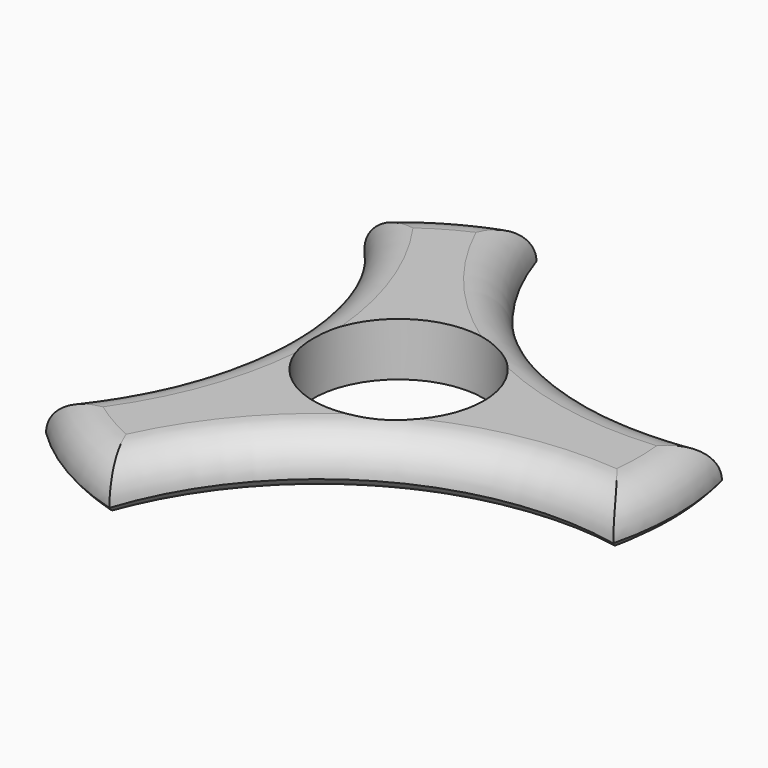
from build123d import *

# Parameters (mm, degrees)
F0_R         = 11.2
F1_DEPTH     = 7
F2_T2_ANGLE  = 120.2325245339
F2_T4_ANGLE  = 67.6545772904
F2_T6_ANGLE  = 120.2325245339
F2_T8_ANGLE  = 67.6545772904
F2_T10_ANGLE = 120.2325245339
F2_T12_ANGLE = 67.6545772904
F3_T2_ANGLE  = 112.9190333921
F3_T4_ANGLE  = 59.7918695457
F3_T6_ANGLE  = 112.9190333921
F3_T8_ANGLE  = 112.9190333921
F3_T10_ANGLE = 59.7918695457
F3_T12_ANGLE = 59.7918694889


# Not quite as in the source:
# - a fillet or chamfer that OpenCascade refuses, or shapes differently, is made with other operations: its cross-section is extruded or revolved along the edge and cut away or added


with BuildPart() as f1:
    # F0 (on Top) → F1 (new body)
    with BuildSketch(Plane.XY):
        with BuildLine():
            ThreePointArc((35.3273925443, 8.9196701012), (7.7000134584, 13.3368145289), (-9.9390353711, 35.0542544434))
            ThreePointArc((-9.9390353711, 35.0542544434), (-18.2180211514, 31.5545382476), (-25.3883571732, 26.1345843422))
            ThreePointArc((-25.3883571732, 26.1345843422), (-15.4000269168, 0), (-25.3883571732, -26.1345843422))
            ThreePointArc((-25.3883571732, -26.1345843422), (-18.2180211514, -31.5545382476), (-9.9390353711, -35.0542544434))
            ThreePointArc((-9.9390353711, -35.0542544434), (7.7000134584, -13.3368145289), (35.3273925443, -8.9196701012))
            ThreePointArc((35.3273925443, -8.9196701012), (36.4360423028, 0), (35.3273925443, 8.9196701012))
        make_face()
        Circle(F0_R, mode=Mode.SUBTRACT)
    extrude(amount=F1_DEPTH)

    # F2: fillet of radius 5 on 6 edges, made by hand

    # F2_s1 → F2_t2 (revolve, cut)
    with BuildSketch(Plane(origin=(0.0960343807, -47.3271104631, 0), x_dir=(0, 0, 1), z_dir=(0.002029158, -0.9999979413, 0))):
        with BuildLine():
            ThreePointArc((2, 11.9884098139), (5.5355339059, 13.452875908), (7, 16.9884098139))
            Line((7, 16.9884098139), (7, 11.9884098139))
            Line((7, 11.9884098139), (2, 11.9884098139))
        make_face()
    revolve(axis=Axis((27.2924583405, -47.2719245092, 7), (0, 0, -1)), revolution_arc=F2_T2_ANGLE, mode=Mode.SUBTRACT)

    # F2_s3 → F2_t4 (revolve, cut)
    with BuildSketch(Plane(origin=(0, 0, 0), x_dir=(0, 0, 1), z_dir=(-0.5566913309, -0.8307194244, 0))):
        with BuildLine():
            ThreePointArc((2, -36.4360423028), (5.5355339059, -34.9715762088), (7, -31.4360423028))
            Line((7, -31.4360423028), (7, -36.4360423028))
            Line((7, -36.4360423028), (2, -36.4360423028))
        make_face()
    revolve(axis=Axis((0, 0, 7), (0, 0, 1)), revolution_arc=F2_T4_ANGLE, mode=Mode.SUBTRACT)

    # F2_s5 → F2_t6 (revolve, cut)
    with BuildSketch(Plane(origin=(40.9384627584, 23.7467234449, 0), x_dir=(0, 0, 1), z_dir=(0.8650090419, 0.501756273, 0))):
        with BuildLine():
            ThreePointArc((2, 11.9884098139), (5.5355339059, 13.452875908), (7, 16.9884098139))
            Line((7, 16.9884098139), (7, 11.9884098139))
            Line((7, 11.9884098139), (2, 11.9884098139))
        make_face()
    revolve(axis=Axis((27.2924583405, 47.2719245092, 7), (0, 0, -1)), revolution_arc=F2_T6_ANGLE, mode=Mode.SUBTRACT)

    # F2_s7 → F2_t8 (revolve, cut)
    with BuildSketch(Plane(origin=(0, 0, 0), x_dir=(0, 0, 1), z_dir=(0.9977697904, -0.0667491225, 0))):
        with BuildLine():
            ThreePointArc((2, -36.4360423028), (5.5355339059, -34.9715762088), (7, -31.4360423028))
            Line((7, -31.4360423028), (7, -36.4360423028))
            Line((7, -36.4360423028), (2, -36.4360423028))
        make_face()
    revolve(axis=Axis((0, 0, 7), (0, 0, 1)), revolution_arc=F2_T8_ANGLE, mode=Mode.SUBTRACT)

    # F2_s9 → F2_t10 (revolve, cut)
    with BuildSketch(Plane(origin=(-41.0344971391, 23.5803870182, 0), x_dir=(0, 0, 1), z_dir=(-0.8670381998, 0.4982416683, 0))):
        with BuildLine():
            ThreePointArc((2, 11.9884098139), (5.5355339059, 13.452875908), (7, 16.9884098139))
            Line((7, 16.9884098139), (7, 11.9884098139))
            Line((7, 11.9884098139), (2, 11.9884098139))
        make_face()
    revolve(axis=Axis((-54.5849166811, 0, 7), (0, 0, -1)), revolution_arc=F2_T10_ANGLE, mode=Mode.SUBTRACT)

    # F2_s11 → F2_t12 (revolve, cut)
    with BuildSketch(Plane(origin=(0, 0, 0), x_dir=(0, 0, 1), z_dir=(-0.4410784595, 0.8974685469, 0))):
        with BuildLine():
            ThreePointArc((2, -36.4360423028), (5.5355339059, -34.9715762088), (7, -31.4360423028))
            Line((7, -31.4360423028), (7, -36.4360423028))
            Line((7, -36.4360423028), (2, -36.4360423028))
        make_face()
    revolve(axis=Axis((0, 0, 7), (0, 0, 1)), revolution_arc=F2_T12_ANGLE, mode=Mode.SUBTRACT)

    # F3: fillet of radius 5 on 6 edges, made by hand

    # F3_s1 → F3_t2 (revolve, cut)
    with BuildSketch(Plane(origin=(-2.8095675604, -45.4094561458, 0), x_dir=(0, 0, 1), z_dir=(-0.0617537733, -0.9980914144, 0))):
        with BuildLine():
            ThreePointArc((0, 13.0253017076), (0.527864045, 10.7892337301), (2, 9.0253017076))
            Line((2, 9.0253017076), (0, 9.0253017076))
            Line((0, 9.0253017076), (0, 13.0253017076))
        make_face()
    revolve(axis=Axis((27.2924583405, -47.2719245092, 0), (0, 0, -1)), revolution_arc=F3_T2_ANGLE, mode=Mode.SUBTRACT)

    # F3_s3 → F3_t4 (revolve, cut)
    with BuildSketch(Plane(origin=(0, 0, 0), x_dir=(0, 0, 1), z_dir=(-0.5015721198, 0.8651158354, 0))):
        with BuildLine():
            ThreePointArc((0, -32.4360271055), (0.5278697087, -34.6721064105), (2.0000202632, -36.4360423028))
            Line((2.0000202632, -36.4360423028), (0, -36.4360423028))
            Line((0, -36.4360423028), (0, -32.4360271055))
        make_face()
    revolve(axis=Axis((0, 0, 0), (0, 0, 1)), revolution_arc=F3_T4_ANGLE, mode=Mode.SUBTRACT)

    # F3_s5 → F3_t6 (revolve, cut)
    with BuildSketch(Plane(origin=(-37.920958814, 25.1378849539, 0), x_dir=(0, 0, 1), z_dir=(-0.8334956335, 0.5525260436, 0))):
        with BuildLine():
            ThreePointArc((0, 13.0253017076), (0.527864045, 10.7892337301), (2, 9.0253017076))
            Line((2, 9.0253017076), (0, 9.0253017076))
            Line((0, 9.0253017076), (0, 13.0253017076))
        make_face()
    revolve(axis=Axis((-54.5849166811, 0, 0), (0, 0, -1)), revolution_arc=F3_T6_ANGLE, mode=Mode.SUBTRACT)

    # F3_s7 → F3_t8 (revolve, cut)
    with BuildSketch(Plane(origin=(40.7305263745, 20.2715711919, 0), x_dir=(0, 0, 1), z_dir=(0.8952494068, 0.4455653707, 0))):
        with BuildLine():
            ThreePointArc((2, 9.0253017076), (0.527864045, 10.7892337301), (0, 13.0253017076))
            Line((0, 13.0253017076), (0, 9.0253017076))
            Line((0, 9.0253017076), (2, 9.0253017076))
        make_face()
    revolve(axis=Axis((27.2924583405, 47.2719245092, 0), (0, 0, -1)), revolution_arc=F3_T8_ANGLE, mode=Mode.SUBTRACT)

    # F3_s9 → F3_t10 (revolve, cut)
    with BuildSketch(Plane(origin=(0, 0, 0), x_dir=(0, 0, 1), z_dir=(0.9999983506, 0.0018162799, 0))):
        with BuildLine():
            ThreePointArc((0, -32.4360271055), (0.5278697087, -34.6721064105), (2.0000202632, -36.4360423028))
            Line((2.0000202632, -36.4360423028), (0, -36.4360423028))
            Line((0, -36.4360423028), (0, -32.4360271055))
        make_face()
    revolve(axis=Axis((0, 0, 0), (0, 0, 1)), revolution_arc=F3_T10_ANGLE, mode=Mode.SUBTRACT)

    # F3_s11 → F3_t12 (revolve, cut)
    with BuildSketch(Plane(origin=(0, 0, 0), x_dir=(0, 0, 1), z_dir=(-0.4984262304, -0.8669321155, 0))):
        with BuildLine():
            ThreePointArc((0, -32.4360271128), (0.527869706, -34.6721064123), (2.0000202535, -36.4360423028))
            Line((2.0000202535, -36.4360423028), (0, -36.4360423028))
            Line((0, -36.4360423028), (0, -32.4360271128))
        make_face()
    revolve(axis=Axis((0, 0, 0), (0, 0, 1)), revolution_arc=F3_T12_ANGLE, mode=Mode.SUBTRACT)


solid = f1.part
